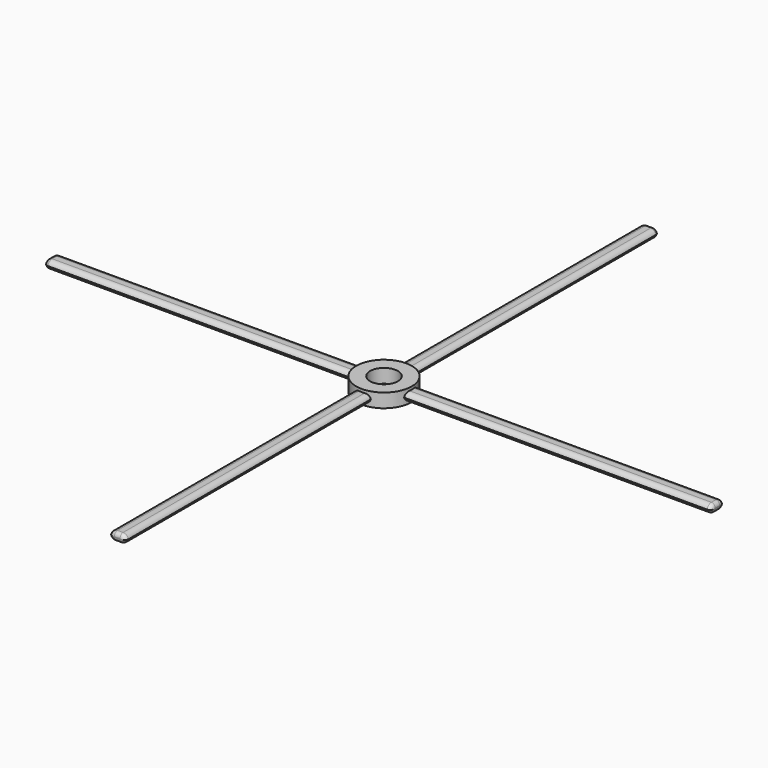
from build123d import *

# Parameters (mm, degrees)
F0_R          = 12.7
F0_R_2        = 6.35
F1_DEPTH      = 6.35
F3_W          = 3.81
F3_H          = 3.81
F5_T4_DEPTH   = 152.984972142
F5_S5_R       = 12.7
F5_T6_DEPTH   = 78
F5_T10_DEPTH  = 152.984972142
F5_S11_R      = 12.7
F5_T12_DEPTH  = 78
F5_T16_DEPTH  = 152.984972142
F5_S17_R      = 12.7
F5_T18_DEPTH  = 78
F5_T22_DEPTH  = 152.984972142
F5_S23_R      = 12.7
F5_T24_DEPTH  = 78
F6_T1_DEPTH   = 2.54
F6_T4_ANGLE   = 175.8184617318
F6_T6_ANGLE   = 175.8184617318
F6_T8_ANGLE   = 175.8184617318
F6_T10_ANGLE  = 175.8184617318
F9_W          = 3.81
F9_H          = 3.81
F11_T4_DEPTH  = 152.984972142
F11_S5_R      = 12.7
F11_T6_DEPTH  = 78
F11_T10_DEPTH = 152.984972142
F11_S11_R     = 12.7
F11_T12_DEPTH = 78
F11_T16_DEPTH = 152.984972142
F11_S17_R     = 12.7
F11_T18_DEPTH = 78
F11_T22_DEPTH = 152.984972142
F11_S23_R     = 12.7
F11_T24_DEPTH = 78
F12_T1_DEPTH  = 2.54
F12_T4_ANGLE  = 175.8184617318
F12_T6_ANGLE  = 175.8184617318
F12_T8_ANGLE  = 175.8184617318
F12_T10_ANGLE = 175.8184617318


# Not quite as in the source:
# - a fillet or chamfer that OpenCascade refuses, or shapes differently, is made with other operations: its cross-section is extruded or revolved along the edge and cut away or added


with BuildPart() as f1:
    # F0 (on Top) → F1 (new body)
    with BuildSketch(Plane.XY):
        Circle(F0_R)
        Circle(F0_R_2, mode=Mode.SUBTRACT)
    extrude(amount=F1_DEPTH)

    # F3 (on offset) → F4 (join, up to the next surface of F1)
    with BuildSketch(Plane.YZ.offset(152.4)):
        with Locations((1.905, 3.175)):
            Rectangle(F3_W, F3_H)
        with Locations((-1.905, 3.175)):
            Rectangle(F3_W, F3_H)
    extrude(until=Until.NEXT, dir=(-1, 0, 0))

    # F5: fillet of radius 2.54 on 4 edges, made by hand


with BuildPart() as f5_tool2:
    # F5_s3 → F5_t4 (new body)
    with BuildSketch(Plane.YZ.offset(158.75)):
        with BuildLine():
            ThreePointArc((-3.81, 2.54), (-3.0660512242, 4.3360512242), (-1.27, 5.08))
            Line((-1.27, 5.08), (-3.81, 5.08))
            Line((-3.81, 5.08), (-3.81, 2.54))
        make_face()
    extrude(amount=-F5_T4_DEPTH)

    # F5_s5 → F5_t6 (cut, symmetric)
    with BuildSketch(Plane.XY.offset(3.8)):
        Circle(F5_S5_R)
    extrude(amount=F5_T6_DEPTH, both=True, mode=Mode.SUBTRACT)


with BuildPart() as f1_1:
    add(f1.part)

    # F5_t1: cut F5_tool2
    add(f5_tool2.part, mode=Mode.SUBTRACT)


with BuildPart() as f5_tool8:
    # F5_s9 → F5_t10 (new body)
    with BuildSketch(Plane.YZ.offset(158.75)):
        with BuildLine():
            ThreePointArc((1.27, 5.08), (3.0660512242, 4.3360512242), (3.81, 2.54))
            Line((3.81, 2.54), (3.81, 5.08))
            Line((3.81, 5.08), (1.27, 5.08))
        make_face()
    extrude(amount=-F5_T10_DEPTH)

    # F5_s11 → F5_t12 (cut, symmetric)
    with BuildSketch(Plane.XY.offset(3.8)):
        Circle(F5_S11_R)
    extrude(amount=F5_T12_DEPTH, both=True, mode=Mode.SUBTRACT)


with BuildPart() as f1_2:
    add(f1_1.part)

    # F5_t7: cut F5_tool8
    add(f5_tool8.part, mode=Mode.SUBTRACT)


with BuildPart() as f5_tool14:
    # F5_s15 → F5_t16 (new body)
    with BuildSketch(Plane.YZ.offset(158.75)):
        with BuildLine():
            ThreePointArc((-1.27, 1.27), (-3.0660512242, 2.0139487758), (-3.81, 3.81))
            Line((-3.81, 3.81), (-3.81, 1.27))
            Line((-3.81, 1.27), (-1.27, 1.27))
        make_face()
    extrude(amount=-F5_T16_DEPTH)

    # F5_s17 → F5_t18 (cut, symmetric)
    with BuildSketch(Plane.XY.offset(2.5)):
        Circle(F5_S17_R)
    extrude(amount=F5_T18_DEPTH, both=True, mode=Mode.SUBTRACT)


with BuildPart() as f1_3:
    add(f1_2.part)

    # F5_t13: cut F5_tool14
    add(f5_tool14.part, mode=Mode.SUBTRACT)


with BuildPart() as f5_tool20:
    # F5_s21 → F5_t22 (new body)
    with BuildSketch(Plane.YZ.offset(158.75)):
        with BuildLine():
            ThreePointArc((1.27, 1.27), (3.0660512242, 2.0139487758), (3.81, 3.81))
            Line((3.81, 3.81), (3.81, 1.27))
            Line((3.81, 1.27), (1.27, 1.27))
        make_face()
    extrude(amount=-F5_T22_DEPTH)

    # F5_s23 → F5_t24 (cut, symmetric)
    with BuildSketch(Plane.XY.offset(2.5)):
        Circle(F5_S23_R)
    extrude(amount=F5_T24_DEPTH, both=True, mode=Mode.SUBTRACT)


with BuildPart() as f1_4:
    add(f1_3.part)

    # F5_t19: cut F5_tool20
    add(f5_tool20.part, mode=Mode.SUBTRACT)

    # F6: fillet of radius 1.778 on 6 edges, made by hand

    # F6_s2 → F6_t1 (cut)
    with BuildSketch(Plane.XZ.offset(-1.27)):
        with BuildLine():
            ThreePointArc((150.622, 5.08), (151.8792358569, 4.5592358569), (152.4, 3.302))
            Line((152.4, 3.302), (152.4, 5.08))
            Line((152.4, 5.08), (150.622, 5.08))
        make_face()
        with BuildLine():
            ThreePointArc((150.622, 1.27), (151.8792358569, 1.7907641431), (152.4, 3.048))
            Line((152.4, 3.048), (152.4, 1.27))
            Line((152.4, 1.27), (150.622, 1.27))
        make_face()
    extrude(amount=F6_T1_DEPTH, mode=Mode.SUBTRACT)

    # F6_s3 → F6_t4 (revolve, cut)
    with BuildSketch(Plane(origin=(0, -0.9861739497, -0.0721006188), x_dir=(1, 0, 0), z_dir=(0, 0.9973380241, 0.0729168406))):
        with BuildLine():
            ThreePointArc((150.622, -6.4324622596), (151.8792358569, -5.9116981165), (152.4, -4.6544622596))
            Line((152.4, -4.6544622596), (152.4, -6.4324622596))
            Line((152.4, -6.4324622596), (150.622, -6.4324622596))
        make_face()
    revolve(axis=Axis((152.4, -1.27, 3.81), (1, 0, 0)), revolution_arc=F6_T4_ANGLE, mode=Mode.SUBTRACT)

    # F6_s5 → F6_t6 (revolve, cut)
    with BuildSketch(Plane.XZ.offset(1.27)):
        with BuildLine():
            ThreePointArc((150.622, 5.08), (151.8792358569, 4.5592358569), (152.4, 3.302))
            Line((152.4, 3.302), (152.4, 5.08))
            Line((152.4, 5.08), (150.622, 5.08))
        make_face()
    revolve(axis=Axis((152.4, -1.27, 2.54), (1, 0, 0)), revolution_arc=F6_T6_ANGLE, mode=Mode.SUBTRACT)

    # F6_s7 → F6_t8 (revolve, cut)
    with BuildSketch(Plane(origin=(0, 1.4479633345, 0.1058627157), x_dir=(1, 0, 0), z_dir=(0, -0.9973380241, -0.0729168406))):
        with BuildLine():
            ThreePointArc((150.622, -0.0993658064), (151.8792358569, 0.4213983366), (152.4, 1.6786341936))
            Line((152.4, 1.6786341936), (152.4, -0.0993658064))
            Line((152.4, -0.0993658064), (150.622, -0.0993658064))
        make_face()
    revolve(axis=Axis((152.4, 1.27, 2.54), (1, 0, 0)), revolution_arc=F6_T8_ANGLE, mode=Mode.SUBTRACT)

    # F6_s9 → F6_t10 (revolve, cut)
    with BuildSketch(Plane.XZ.offset(-1.27)):
        with BuildLine():
            ThreePointArc((150.622, 1.27), (151.8792358569, 1.7907641431), (152.4, 3.048))
            Line((152.4, 3.048), (152.4, 1.27))
            Line((152.4, 1.27), (150.622, 1.27))
        make_face()
    revolve(axis=Axis((152.4, 1.27, 3.81), (1, 0, 0)), revolution_arc=F6_T10_ANGLE, mode=Mode.SUBTRACT)

    # F7: F1 across plane


with BuildPart() as f1_5:
    add(f1_4.part)
    add(f1_4.part.mirror(Plane.YZ))

    # F9 (on offset) → F10 (join, up to the next surface of F1)
    with BuildSketch(Plane.XZ.offset(-152.4)):
        with Locations((1.905, 3.175)):
            Rectangle(F9_W, F9_H)
        with Locations((-1.905, 3.175)):
            Rectangle(F9_W, F9_H)
    extrude(until=Until.NEXT)

    # F11: fillet of radius 2.54 on 4 edges, made by hand


with BuildPart() as f11_tool2:
    # F11_s3 → F11_t4 (new body)
    with BuildSketch(Plane.XZ.offset(-158.75)):
        with BuildLine():
            ThreePointArc((1.27, 5.08), (3.0660512242, 4.3360512242), (3.81, 2.54))
            Line((3.81, 2.54), (3.81, 5.08))
            Line((3.81, 5.08), (1.27, 5.08))
        make_face()
    extrude(amount=F11_T4_DEPTH)

    # F11_s5 → F11_t6 (cut, symmetric)
    with BuildSketch(Plane.XY.offset(3.8)):
        Circle(F11_S5_R)
    extrude(amount=F11_T6_DEPTH, both=True, mode=Mode.SUBTRACT)


with BuildPart() as f1_6:
    add(f1_5.part)

    # F11_t1: cut F11_tool2
    add(f11_tool2.part, mode=Mode.SUBTRACT)


with BuildPart() as f11_tool8:
    # F11_s9 → F11_t10 (new body)
    with BuildSketch(Plane.XZ.offset(-158.75)):
        with BuildLine():
            ThreePointArc((1.27, 1.27), (3.0660512242, 2.0139487758), (3.81, 3.81))
            Line((3.81, 3.81), (3.81, 1.27))
            Line((3.81, 1.27), (1.27, 1.27))
        make_face()
    extrude(amount=F11_T10_DEPTH)

    # F11_s11 → F11_t12 (cut, symmetric)
    with BuildSketch(Plane.XY.offset(2.5)):
        Circle(F11_S11_R)
    extrude(amount=F11_T12_DEPTH, both=True, mode=Mode.SUBTRACT)


with BuildPart() as f1_7:
    add(f1_6.part)

    # F11_t7: cut F11_tool8
    add(f11_tool8.part, mode=Mode.SUBTRACT)


with BuildPart() as f11_tool14:
    # F11_s15 → F11_t16 (new body)
    with BuildSketch(Plane.XZ.offset(-158.75)):
        with BuildLine():
            ThreePointArc((-1.27, 5.08), (-3.0660512242, 4.3360512242), (-3.81, 2.54))
            Line((-3.81, 2.54), (-3.81, 5.08))
            Line((-3.81, 5.08), (-1.27, 5.08))
        make_face()
    extrude(amount=F11_T16_DEPTH)

    # F11_s17 → F11_t18 (cut, symmetric)
    with BuildSketch(Plane.XY.offset(3.8)):
        Circle(F11_S17_R)
    extrude(amount=F11_T18_DEPTH, both=True, mode=Mode.SUBTRACT)


with BuildPart() as f1_8:
    add(f1_7.part)

    # F11_t13: cut F11_tool14
    add(f11_tool14.part, mode=Mode.SUBTRACT)


with BuildPart() as f11_tool20:
    # F11_s21 → F11_t22 (new body)
    with BuildSketch(Plane.XZ.offset(-158.75)):
        with BuildLine():
            ThreePointArc((-3.81, 3.81), (-3.0660512242, 2.0139487758), (-1.27, 1.27))
            Line((-1.27, 1.27), (-3.81, 1.27))
            Line((-3.81, 1.27), (-3.81, 3.81))
        make_face()
    extrude(amount=F11_T22_DEPTH)

    # F11_s23 → F11_t24 (cut, symmetric)
    with BuildSketch(Plane.XY.offset(2.5)):
        Circle(F11_S23_R)
    extrude(amount=F11_T24_DEPTH, both=True, mode=Mode.SUBTRACT)


with BuildPart() as f1_9:
    add(f1_8.part)

    # F11_t19: cut F11_tool20
    add(f11_tool20.part, mode=Mode.SUBTRACT)

    # F12: fillet of radius 1.778 on 6 edges, made by hand

    # F12_s2 → F12_t1 (cut)
    with BuildSketch(Plane.YZ.offset(-1.27)):
        with BuildLine():
            ThreePointArc((150.622, 5.08), (151.8792358569, 4.5592358569), (152.4, 3.302))
            Line((152.4, 3.302), (152.4, 5.08))
            Line((152.4, 5.08), (150.622, 5.08))
        make_face()
        with BuildLine():
            ThreePointArc((150.622, 1.27), (151.8792358569, 1.7907641431), (152.4, 3.048))
            Line((152.4, 3.048), (152.4, 1.27))
            Line((152.4, 1.27), (150.622, 1.27))
        make_face()
    extrude(amount=F12_T1_DEPTH, mode=Mode.SUBTRACT)

    # F12_s3 → F12_t4 (revolve, cut)
    with BuildSketch(Plane.YZ.offset(-1.27)):
        with BuildLine():
            ThreePointArc((150.622, 1.27), (151.8792358569, 1.7907641431), (152.4, 3.048))
            Line((152.4, 3.048), (152.4, 1.27))
            Line((152.4, 1.27), (150.622, 1.27))
        make_face()
    revolve(axis=Axis((-1.27, 152.4, 3.81), (0, 1, 0)), revolution_arc=F12_T4_ANGLE, mode=Mode.SUBTRACT)

    # F12_s5 → F12_t6 (revolve, cut)
    with BuildSketch(Plane(origin=(-1.4479633345, 0, 0.1058627157), x_dir=(0, 1, 0), z_dir=(0.9973380241, 0, -0.0729168406))):
        with BuildLine():
            ThreePointArc((150.622, -0.0993658064), (151.8792358569, 0.4213983366), (152.4, 1.6786341936))
            Line((152.4, 1.6786341936), (152.4, -0.0993658064))
            Line((152.4, -0.0993658064), (150.622, -0.0993658064))
        make_face()
    revolve(axis=Axis((-1.27, 152.4, 2.54), (0, 1, 0)), revolution_arc=F12_T6_ANGLE, mode=Mode.SUBTRACT)

    # F12_s7 → F12_t8 (revolve, cut)
    with BuildSketch(Plane(origin=(0.9861739497, 0, -0.0721006188), x_dir=(0, 1, 0), z_dir=(-0.9973380241, 0, 0.0729168406))):
        with BuildLine():
            ThreePointArc((150.622, -6.4324622596), (151.8792358569, -5.9116981165), (152.4, -4.6544622596))
            Line((152.4, -4.6544622596), (152.4, -6.4324622596))
            Line((152.4, -6.4324622596), (150.622, -6.4324622596))
        make_face()
    revolve(axis=Axis((1.27, 152.4, 3.81), (0, 1, 0)), revolution_arc=F12_T8_ANGLE, mode=Mode.SUBTRACT)

    # F12_s9 → F12_t10 (revolve, cut)
    with BuildSketch(Plane.YZ.offset(1.27)):
        with BuildLine():
            ThreePointArc((150.622, 5.08), (151.8792358569, 4.5592358569), (152.4, 3.302))
            Line((152.4, 3.302), (152.4, 5.08))
            Line((152.4, 5.08), (150.622, 5.08))
        make_face()
    revolve(axis=Axis((1.27, 152.4, 2.54), (0, 1, 0)), revolution_arc=F12_T10_ANGLE, mode=Mode.SUBTRACT)

    # F13: F1 across plane


with BuildPart() as f1_10:
    add(f1_9.part)
    add(f1_9.part.mirror(Plane.XZ))


with BuildPart() as f14_1:
    # F14: copy of F1
    add(f1_10.part)


solid = Compound([f1_10.part, f14_1.part])
